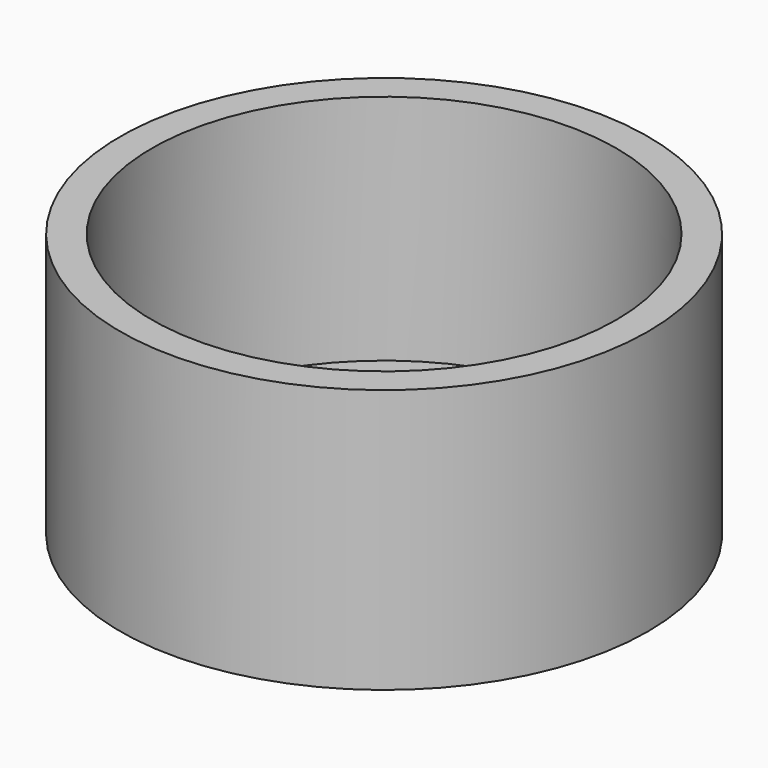
from build123d import *

# Parameters (mm, degrees)
F2_R     = 635
F3_DEPTH = 635
F4_T     = -76.2


# Not quite as in the source:
# - a variable given as a bare number and used for a length is read in inches; the dataset says mm whatever the document's units were


with BuildPart() as f3:
    # F2 (on Top) → F3 (new body)
    with BuildSketch(Plane.XY):
        Circle(F2_R)
    extrude(amount=F3_DEPTH)

    # F4
    f4_openings = [f3.faces().sort_by_distance(p)[0] for p in [
        (0, 0, 635),
    ]]
    offset(amount=F4_T, openings=f4_openings)


solid = f3.part
